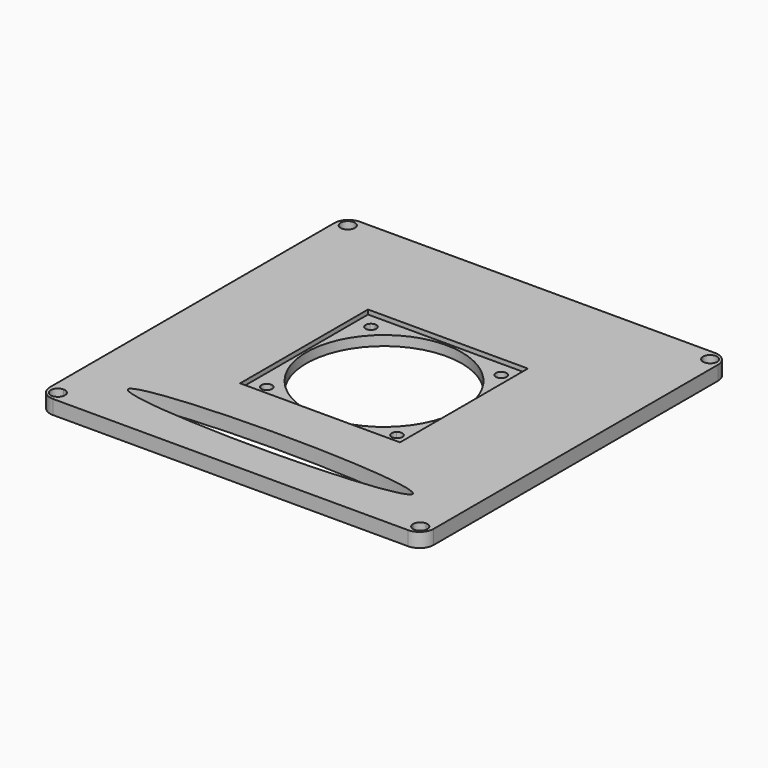
from build123d import *

# Parameters (mm, degrees)
F0_W             = 137.16
F0_H             = 137.16
F1_DEPTH         = 5.08
F2_R             = 5.08
F3_R             = 27.78125
F4_DEPTH         = 5.08
F5_W             = 57.15
F5_H             = 57.15
F6_DEPTH         = 1.5875
F8_DEPTH         = 3.4925
F8_COPIES_COUNT  = 4
F11_DEPTH        = 1.27
F11_COPIES_COUNT = 4
F13_DEPTH        = 5.08
F15_DEPTH        = 5.08


# Not quite as in the source:
# - a pattern or mirror of a feature is missing from the dataset's text; its kind, count and spacing are read off the source's solid


with BuildPart() as f1:
    # F0 (on Top) → F1 (new body)
    with BuildSketch(Plane.XY):
        Rectangle(F0_W, F0_H)
    extrude(amount=F1_DEPTH)

    # F2
    f2_edges = [f1.edges().sort_by_distance(p)[0] for p in [
        (-68.58, -68.58, 2.54),
        (68.58, -68.58, 2.54),
        (68.58, 68.58, 2.54),
        (-68.58, 68.58, 2.54),
    ]]
    fillet(f2_edges, radius=F2_R)

    # F3 (on face) → F4 (cut, through all)
    with BuildSketch(Plane.XY.offset(5.08)):
        Circle(F3_R)
    extrude(amount=-F4_DEPTH, mode=Mode.SUBTRACT)

    # F5 (on face) → F6 (cut)
    with BuildSketch(Plane.XY.offset(5.08)):
        Rectangle(F5_W, F5_H)
    extrude(amount=-F6_DEPTH, mode=Mode.SUBTRACT)

    # F7 (on face) → F8 (cut, through all)
    with BuildSketch(Plane.XY.offset(3.4925)):
        with BuildLine():
            Line((21.9296104704, 21.9296104704), (24.6236873067, 24.6236873067))
            ThreePointArc((24.6236873067, 24.6236873067), (21.9296104704, 24.6236873067), (21.9296104704, 21.9296104704))
        make_face()
        with BuildLine():
            ThreePointArc((25.1816488886, 23.2766488886), (25.036639398, 24.0056608272), (24.6236873067, 24.6236873067))
            Line((24.6236873067, 24.6236873067), (21.9296104704, 21.9296104704))
            ThreePointArc((21.9296104704, 21.9296104704), (24.0056608272, 21.5166583791), (25.1816488886, 23.2766488886))
        make_face()
    f8 = extrude(amount=-F8_DEPTH, mode=Mode.SUBTRACT)

    # F8_copies: F8 ×4 about axis
    f8_copies_axis = Axis((0, 0, 0), (0, 0, 1))
    for i in range(1, F8_COPIES_COUNT):
        add(f8.rotate(f8_copies_axis, i * 360 / F8_COPIES_COUNT), mode=Mode.SUBTRACT)

    # F10 (on face) → F11 (cut)
    with BuildSketch(Plane(origin=(0, 0, 0), x_dir=(1, 0, 0), z_dir=(0, 0, -1))):
        Polygon((27.0866488886, 23.2766488886), (25.1816488886, 26.576205677), (21.3716488886, 26.576205677), (19.4666488886, 23.2766488886), (21.3716488886, 19.9770921002), (25.1816488886, 19.9770921002), align=None)
    f11 = extrude(amount=-F11_DEPTH, mode=Mode.SUBTRACT)

    # F11_copies: F11 ×4 about axis
    f11_copies_axis = Axis((0, 0, 0), (0, 0, 1))
    for i in range(1, F11_COPIES_COUNT):
        add(f11.rotate(f11_copies_axis, i * 360 / F11_COPIES_COUNT), mode=Mode.SUBTRACT)

    # F12 (on face) → F13 (cut, through all)
    with BuildSketch(Plane.XY.offset(5.08)):
        with BuildLine():
            Line((-64.77, 64.77), (-62.23, 64.77))
            ThreePointArc((-62.23, 64.77), (-66.5660512242, 66.5660512242), (-64.77, 62.23))
            Line((-64.77, 62.23), (-64.77, 64.77))
        make_face()
        with BuildLine():
            ThreePointArc((-64.77, 62.23), (-62.9739487758, 62.9739487758), (-62.23, 64.77))
            Line((-62.23, 64.77), (-64.77, 64.77))
            Line((-64.77, 64.77), (-64.77, 62.23))
        make_face()
        with BuildLine():
            Line((-64.77, -64.77), (-64.77, -62.23))
            ThreePointArc((-64.77, -62.23), (-66.5660512242, -66.5660512242), (-62.23, -64.77))
            Line((-62.23, -64.77), (-64.77, -64.77))
        make_face()
        with BuildLine():
            ThreePointArc((-62.23, -64.77), (-62.9739487758, -62.9739487758), (-64.77, -62.23))
            Line((-64.77, -62.23), (-64.77, -64.77))
            Line((-64.77, -64.77), (-62.23, -64.77))
        make_face()
        with BuildLine():
            ThreePointArc((67.31, -64.77), (66.5660512242, -62.9739487758), (64.77, -62.23))
            Line((64.77, -62.23), (64.77, -64.77))
            Line((64.77, -64.77), (62.23, -64.77))
            ThreePointArc((62.23, -64.77), (64.77, -67.31), (67.31, -64.77))
        make_face()
        with BuildLine():
            Line((64.77, -64.77), (64.77, -62.23))
            ThreePointArc((64.77, -62.23), (62.9739487758, -62.9739487758), (62.23, -64.77))
            Line((62.23, -64.77), (64.77, -64.77))
        make_face()
        with BuildLine():
            Line((64.77, 64.77), (62.23, 64.77))
            ThreePointArc((62.23, 64.77), (62.9739487758, 62.9739487758), (64.77, 62.23))
            Line((64.77, 62.23), (64.77, 64.77))
        make_face()
        with BuildLine():
            ThreePointArc((67.31, 64.77), (64.77, 67.31), (62.23, 64.77))
            Line((62.23, 64.77), (64.77, 64.77))
            Line((64.77, 64.77), (64.77, 62.23))
            ThreePointArc((64.77, 62.23), (66.5660512242, 62.9739487758), (67.31, 64.77))
        make_face()
    extrude(amount=-F13_DEPTH, mode=Mode.SUBTRACT)

    # F14 (on face) → F15 (cut, through all)
    with BuildSketch(Plane.XY.offset(5.08)):
        with BuildLine():
            add(Edge.make_bspline(
                [(50.8, -50.8), (50.8, -42.0011818976), (-25.4, -46.4005909488), (-101.6, -50.8), (-25.4, -55.1994090512), (50.8, -59.5988181024), (50.8, -50.8)],
                knots=[0, 0, 0, 2.0943951024, 2.0943951024, 4.1887902048, 4.1887902048, 6.2831853072, 6.2831853072, 6.2831853072], degree=2, weights=[1, 0.5, 1, 0.5, 1, 0.5, 1]))
        make_face()
    extrude(amount=-F15_DEPTH, mode=Mode.SUBTRACT)


solid = f1.part
